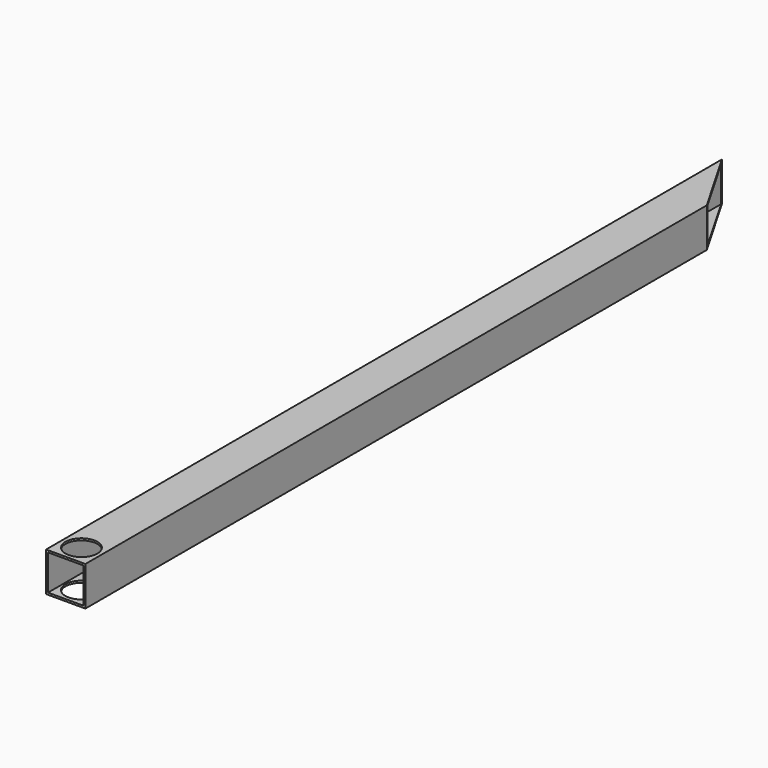
from build123d import *

# Parameters (mm, degrees)
F0_W        = 50.8
F0_H        = 50.8
F1_DEPTH    = 546.1
F2_T        = -2.54
F3_T1_DEPTH = 506.0659394114
F5_D        = 41.275


# Not quite as in the source:
# - a fillet or chamfer that OpenCascade refuses, or shapes differently, is made with other operations: its cross-section is extruded or revolved along the edge and cut away or added


with BuildPart() as f1:
    # F0 (on Front) → F1 (new body, symmetric)
    with BuildSketch(Plane.XZ):
        Rectangle(F0_W, F0_H)
    extrude(amount=F1_DEPTH, both=True)

    # F2
    f2_openings = [f1.faces().sort_by_distance(p)[0] for p in [
        (0, -546.1, 0),
        (0, 546.1, 0),
    ]]
    offset(amount=F2_T, openings=f2_openings)

    # F3: chamfer of 50.8 x 87.9881810245 on 1 edges, made by hand

    # F3_s2 → F3_t1 (cut)
    with BuildSketch(Plane.XY.offset(-253.0329697057)):
        Polygon((25.4, 458.1118189755), (-25.4, 546.1), (25.4, 546.1), align=None)
    extrude(amount=F3_T1_DEPTH, mode=Mode.SUBTRACT)

    # F5 (through all)
    with Locations(Plane.XY.offset(25.4)):
        with Locations((0, -520.7)):
            Hole(F5_D / 2)


solid = f1.part
